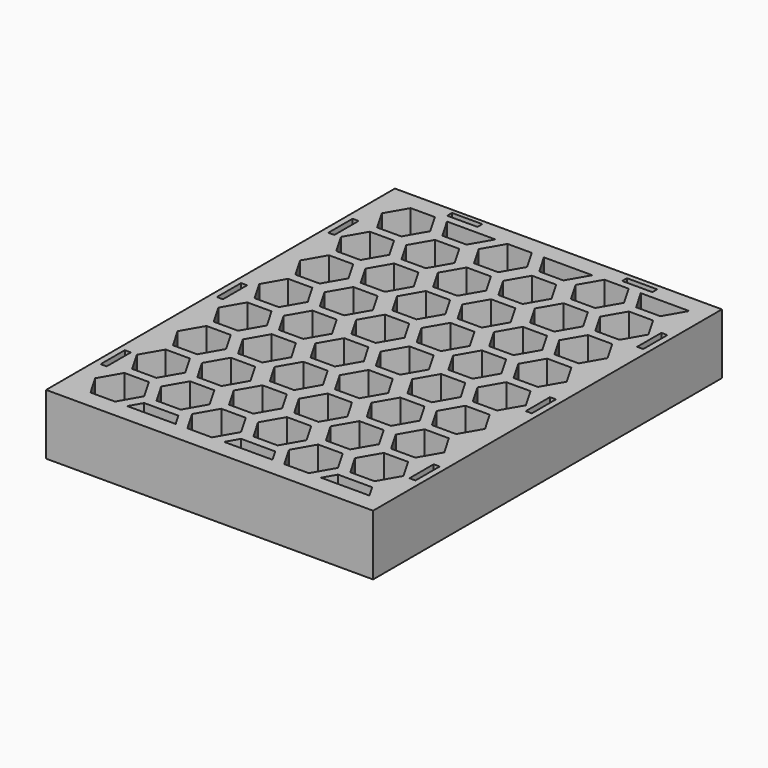
from build123d import *

# Parameters (mm, degrees)
F0_W     = 129.54
F0_H     = 179.07
F1_DEPTH = 25.4
F2_DEPTH = 25.4
F3_DEPTH = 25.4
F5_DEPTH = 25.4
F6_DEPTH = 25.4
F7_W     = 2.54
F7_H     = 12.7
F7_W_2   = 12.7
F7_H_2   = 2.54
F8_DEPTH = 7.62


# Not quite as in the source:
# - a feature names something its author has since deleted; it is built from what else it names


with BuildPart() as f1:
    # F0 (on Top) → F1 (new body)
    with BuildSketch(Plane.XY):
        with Locations((-1.3964310432, 21.6441547314)):
            Rectangle(F0_W, F0_H)
        Polygon((-62.5745659385, -51.3775706631), (-57.4400322633, -42.4842973522), (-47.1709648156, -42.484297296), (-42.0364310432, -51.3775705508), (-47.1709647184, -60.2708438618), (-57.440032166, -60.2708439179), align=None, mode=Mode.SUBTRACT)
        Polygon((-42.0364310432, -60.2708453796), (-39.0470681494, -55.0931169001), (-24.7057939935, -55.0931168217), (-21.7164310432, -60.2708452686), align=None, mode=Mode.SUBTRACT)
        Polygon((-21.9345659385, -51.3775720702), (-16.8000322633, -42.4842987593), (-6.5309648156, -42.4842987032), (-1.3964310432, -51.377571958), (-6.5309647184, -60.2708452689), (-16.800032166, -60.270845325), align=None, mode=Mode.SUBTRACT)
        Polygon((-42.0364310432, -42.4842988139), (-36.9564310912, -33.6854806837), (-26.7964310912, -33.6854806282), (-21.7164310432, -42.4842987029), (-26.7964309951, -51.2831168331), (-36.9564309951, -51.2831168886), align=None, mode=Mode.SUBTRACT)
        Polygon((-21.7164310432, -29.8754806837), (-16.6364310912, -21.0766625535), (-6.4764310912, -21.076662498), (-1.3964310432, -29.8754805727), (-6.4764309951, -38.6742987029), (-16.6364309951, -38.6742987584), align=None, mode=Mode.SUBTRACT)
        Polygon((-42.0364310432, -21.076662609), (-36.9564310912, -12.2778444788), (-26.7964310912, -12.2778444233), (-21.7164310432, -21.076662498), (-26.7964309951, -29.8754806282), (-36.9564309951, -29.8754806837), align=None, mode=Mode.SUBTRACT)
        Polygon((-42.0364310432, 0.3309735959), (-36.9564310912, 9.1297917261), (-26.7964310912, 9.1297917816), (-21.7164310432, 0.3309737069), (-26.7964309951, -8.4678444233), (-36.9564309951, -8.4678444788), align=None, mode=Mode.SUBTRACT)
        Polygon((-21.7164310432, -8.4678444788), (-16.6364310912, 0.3309736514), (-6.4764310912, 0.3309737069), (-1.3964310432, -8.4678443678), (-6.4764309951, -17.266662498), (-16.6364309951, -17.2666625535), align=None, mode=Mode.SUBTRACT)
        Polygon((-42.0364310432, 21.7386098008), (-36.9564310912, 30.537427931), (-26.7964310912, 30.5374279865), (-21.7164310432, 21.7386099118), (-26.7964309951, 12.9397917816), (-36.9564309951, 12.9397917261), align=None, mode=Mode.SUBTRACT)
        Polygon((-21.7164310432, 12.9397917261), (-16.6364310912, 21.7386098563), (-6.4764310912, 21.7386099118), (-1.3964310432, 12.9397918371), (-6.4764309951, 4.1409737069), (-16.6364309951, 4.1409736514), align=None, mode=Mode.SUBTRACT)
        Polygon((-1.3964310432, -60.2708452686), (1.5929318789, -55.0931168053), (15.9342060348, -55.0931168053), (18.9235689568, -60.2708452686), align=None, mode=Mode.SUBTRACT)
        Polygon((18.7054340615, -51.3775719857), (23.8399677854, -42.4842987029), (34.109035233, -42.4842987029), (39.2435689568, -51.3775719857), (34.109035233, -60.2708452686), (23.8399677854, -60.2708452686), align=None, mode=Mode.SUBTRACT)
        Polygon((-1.3964310432, -42.4842987029), (3.6835689568, -33.6854806004), (13.8435689568, -33.6854806004), (18.9235689568, -42.4842987029), (13.8435689568, -51.2831168053), (3.6835689568, -51.2831168053), align=None, mode=Mode.SUBTRACT)
        Polygon((18.9235689568, -29.8754806004), (24.0035689568, -21.076662498), (34.1635689568, -21.076662498), (39.2435689568, -29.8754806004), (34.1635689568, -38.6742987029), (24.0035689568, -38.6742987029), align=None, mode=Mode.SUBTRACT)
        Polygon((39.2435689568, -60.2708452686), (42.2329318789, -55.0931168053), (56.5742060348, -55.0931168053), (59.5635689568, -60.2708452686), align=None, mode=Mode.SUBTRACT)
        Polygon((-1.3964310432, -21.076662498), (3.6835689568, -12.2778443955), (13.8435689568, -12.2778443955), (18.9235689568, -21.076662498), (13.8435689568, -29.8754806004), (3.6835689568, -29.8754806004), align=None, mode=Mode.SUBTRACT)
        Polygon((-1.3964310432, 0.3309737069), (3.6835689568, 9.1297918094), (13.8435689568, 9.1297918094), (18.9235689568, 0.3309737069), (13.8435689568, -8.4678443955), (3.6835689568, -8.4678443955), align=None, mode=Mode.SUBTRACT)
        Polygon((18.9235689568, -8.4678443955), (24.0035689568, 0.3309737069), (34.1635689568, 0.3309737069), (39.2435689568, -8.4678443955), (34.1635689568, -17.266662498), (24.0035689568, -17.266662498), align=None, mode=Mode.SUBTRACT)
        Polygon((-1.3964310432, 21.7386099118), (3.6835689568, 30.5374280143), (13.8435689568, 30.5374280143), (18.9235689568, 21.7386099118), (13.8435689568, 12.9397918094), (3.6835689568, 12.9397918094), align=None, mode=Mode.SUBTRACT)
        Polygon((18.9235689568, 12.9397918094), (24.0035689568, 21.7386099118), (34.1635689568, 21.7386099118), (39.2435689568, 12.9397918094), (34.1635689568, 4.1409737069), (24.0035689568, 4.1409737069), align=None, mode=Mode.SUBTRACT)
        Polygon((-42.0364310432, 43.1462460057), (-36.9564310912, 51.9450641359), (-26.7964310912, 51.9450641914), (-21.7164310432, 43.1462461167), (-26.7964309951, 34.3474279865), (-36.9564309951, 34.347427931), align=None, mode=Mode.SUBTRACT)
        Polygon((-21.7164310432, 34.347427931), (-16.6364310912, 43.1462460612), (-6.4764310912, 43.1462461167), (-1.3964310432, 34.347428042), (-6.4764309951, 25.5486099118), (-16.6364309951, 25.5486098563), align=None, mode=Mode.SUBTRACT)
        Polygon((-42.0364310432, 64.5538822106), (-36.9564310912, 73.3527003408), (-26.7964310912, 73.3527003963), (-21.7164310432, 64.5538823216), (-26.7964309951, 55.7550641914), (-36.9564309951, 55.7550641359), align=None, mode=Mode.SUBTRACT)
        Polygon((-21.7164310432, 55.7550641359), (-16.6364310912, 64.5538822661), (-6.4764310912, 64.5538823216), (-1.3964310432, 55.7550642469), (-6.4764309951, 46.9562461167), (-16.6364309951, 46.9562460612), align=None, mode=Mode.SUBTRACT)
        Polygon((-62.3564310432, 98.5703361507), (-57.2764318716, 107.3691547314), (-47.1164318716, 107.369155688), (-42.0364310432, 98.5703380639), (-47.1164302147, 89.7715194831), (-57.2764302147, 89.7715185265), align=None, mode=Mode.SUBTRACT)
        Polygon((-42.0364310432, 85.9615184155), (-36.9564310912, 94.7603365457), (-26.7964310912, 94.7603366012), (-21.7164310432, 85.9615185265), (-26.7964309951, 77.1627003963), (-36.9564309951, 77.1627003408), align=None, mode=Mode.SUBTRACT)
        Polygon((-21.7164310432, 77.1627003408), (-16.6364310912, 85.961518471), (-6.4764310912, 85.9615185265), (-1.3964310432, 77.1627004518), (-6.4764309951, 68.3638823216), (-16.6364309951, 68.3638822661), align=None, mode=Mode.SUBTRACT)
        Polygon((-36.9564309951, 98.5703365457), (-42.0364310432, 107.3691546204), (-21.7164310432, 107.3691547314), (-26.7964309951, 98.5703366012), align=None, mode=Mode.SUBTRACT)
        Polygon((-21.7164310432, 98.5703365457), (-16.6364310912, 107.3691546759), (-6.4764310912, 107.3691547314), (-1.3964310432, 98.5703366567), (-6.4764309951, 89.7715185265), (-16.6364309951, 89.771518471), align=None, mode=Mode.SUBTRACT)
        Polygon((-1.3964310432, 43.1462461167), (3.6835689568, 51.9450642192), (13.8435689568, 51.9450642192), (18.9235689568, 43.1462461167), (13.8435689568, 34.3474280143), (3.6835689568, 34.3474280143), align=None, mode=Mode.SUBTRACT)
        Polygon((18.9235689568, 34.3474280143), (24.0035689568, 43.1462461167), (34.1635689568, 43.1462461167), (39.2435689568, 34.3474280143), (34.1635689568, 25.5486099118), (24.0035689568, 25.5486099118), align=None, mode=Mode.SUBTRACT)
        Polygon((-1.3964310432, 64.5538823216), (3.6835689568, 73.3527004241), (13.8435689568, 73.3527004241), (18.9235689568, 64.5538823216), (13.8435689568, 55.7550642192), (3.6835689568, 55.7550642192), align=None, mode=Mode.SUBTRACT)
        Polygon((18.9235689568, 55.7550642192), (24.0035689568, 64.5538823216), (34.1635689568, 64.5538823216), (39.2435689568, 55.7550642192), (34.1635689568, 46.9562461167), (24.0035689568, 46.9562461167), align=None, mode=Mode.SUBTRACT)
        Polygon((-1.3964310432, 85.9615185265), (3.6835689568, 94.760336629), (13.8435689568, 94.760336629), (18.9235689568, 85.9615185265), (13.8435689568, 77.1627004241), (3.6835689568, 77.1627004241), align=None, mode=Mode.SUBTRACT)
        Polygon((18.9235689568, 77.1627004241), (24.0035689568, 85.9615185265), (34.1635689568, 85.9615185265), (39.2435689568, 77.1627004241), (34.1635689568, 68.3638823216), (24.0035689568, 68.3638823216), align=None, mode=Mode.SUBTRACT)
        Polygon((3.6835689568, 98.570336629), (-1.3964310432, 107.3691547314), (18.9235689568, 107.3691547314), (13.8435689568, 98.570336629), align=None, mode=Mode.SUBTRACT)
        Polygon((18.9235689568, 98.570336629), (24.0035689568, 107.3691547314), (34.1635689568, 107.3691547314), (39.2435689568, 98.570336629), (34.1635689568, 89.7715185265), (24.0035689568, 89.7715185265), align=None, mode=Mode.SUBTRACT)
        Polygon((44.3235689568, 98.570336629), (39.2435689568, 107.3691547314), (59.5635689568, 107.3691547314), (54.4835689568, 98.570336629), align=None, mode=Mode.SUBTRACT)
        Polygon((34.109035233, -42.4842987029), (23.8399677854, -42.4842987029), (18.7054340615, -51.3775719857), (23.8399677854, -60.2708452686), (34.109035233, -60.2708452686), (39.2435689568, -51.3775719857), align=None)
        Polygon((-6.5309648156, -42.4842987032), (-16.8000322633, -42.4842987593), (-21.9345659385, -51.3775720702), (-16.800032166, -60.270845325), (-6.5309647184, -60.2708452689), (-1.3964310432, -51.377571958), align=None)
        Polygon((-47.1709648156, -42.484297296), (-57.4400322633, -42.4842973522), (-62.5745659385, -51.3775706631), (-57.440032166, -60.2708439179), (-47.1709647184, -60.2708438618), (-42.0364310432, -51.3775705508), align=None)
        Polygon((-26.7964310912, 51.9450641914), (-36.9564310912, 51.9450641359), (-42.0364310432, 43.1462460057), (-36.9564309951, 34.347427931), (-26.7964309951, 34.3474279865), (-21.7164310432, 43.1462461167), align=None)
        Polygon((-6.4764310912, 43.1462461167), (-16.6364310912, 43.1462460612), (-21.7164310432, 34.347427931), (-16.6364309951, 25.5486098563), (-6.4764309951, 25.5486099118), (-1.3964310432, 34.347428042), align=None)
        Polygon((-6.4764310912, 21.7386099118), (-16.6364310912, 21.7386098563), (-21.7164310432, 12.9397917261), (-16.6364309951, 4.1409736514), (-6.4764309951, 4.1409737069), (-1.3964310432, 12.9397918371), align=None)
        Polygon((-6.4764310912, 0.3309737069), (-16.6364310912, 0.3309736514), (-21.7164310432, -8.4678444788), (-16.6364309951, -17.2666625535), (-6.4764309951, -17.266662498), (-1.3964310432, -8.4678443678), align=None)
        Polygon((-26.7964310912, -12.2778444233), (-36.9564310912, -12.2778444788), (-42.0364310432, -21.076662609), (-36.9564309951, -29.8754806837), (-26.7964309951, -29.8754806282), (-21.7164310432, -21.076662498), align=None)
        Polygon((-6.4764310912, -21.076662498), (-16.6364310912, -21.0766625535), (-21.7164310432, -29.8754806837), (-16.6364309951, -38.6742987584), (-6.4764309951, -38.6742987029), (-1.3964310432, -29.8754805727), align=None)
        Polygon((-26.7964310912, -33.6854806282), (-36.9564310912, -33.6854806837), (-42.0364310432, -42.4842988139), (-36.9564309951, -51.2831168886), (-26.7964309951, -51.2831168331), (-21.7164310432, -42.4842987029), align=None)
        Polygon((13.8435689568, -12.2778443955), (3.6835689568, -12.2778443955), (-1.3964310432, -21.076662498), (3.6835689568, -29.8754806004), (13.8435689568, -29.8754806004), (18.9235689568, -21.076662498), align=None)
        Polygon((13.8435689568, 9.1297918094), (3.6835689568, 9.1297918094), (-1.3964310432, 0.3309737069), (3.6835689568, -8.4678443955), (13.8435689568, -8.4678443955), (18.9235689568, 0.3309737069), align=None)
        Polygon((34.1635689568, 0.3309737069), (24.0035689568, 0.3309737069), (18.9235689568, -8.4678443955), (24.0035689568, -17.266662498), (34.1635689568, -17.266662498), (39.2435689568, -8.4678443955), align=None)
        Polygon((34.1635689568, -21.076662498), (24.0035689568, -21.076662498), (18.9235689568, -29.8754806004), (24.0035689568, -38.6742987029), (34.1635689568, -38.6742987029), (39.2435689568, -29.8754806004), align=None)
        Polygon((34.1635689568, 21.7386099118), (24.0035689568, 21.7386099118), (18.9235689568, 12.9397918094), (24.0035689568, 4.1409737069), (34.1635689568, 4.1409737069), (39.2435689568, 12.9397918094), align=None)
        Polygon((13.8435689568, 30.5374280143), (3.6835689568, 30.5374280143), (-1.3964310432, 21.7386099118), (3.6835689568, 12.9397918094), (13.8435689568, 12.9397918094), (18.9235689568, 21.7386099118), align=None)
        Polygon((34.1635689568, 43.1462461167), (24.0035689568, 43.1462461167), (18.9235689568, 34.3474280143), (24.0035689568, 25.5486099118), (34.1635689568, 25.5486099118), (39.2435689568, 34.3474280143), align=None)
        Polygon((13.8435689568, 51.9450642192), (3.6835689568, 51.9450642192), (-1.3964310432, 43.1462461167), (3.6835689568, 34.3474280143), (13.8435689568, 34.3474280143), (18.9235689568, 43.1462461167), align=None)
        Polygon((34.1635689568, 64.5538823216), (24.0035689568, 64.5538823216), (18.9235689568, 55.7550642192), (24.0035689568, 46.9562461167), (34.1635689568, 46.9562461167), (39.2435689568, 55.7550642192), align=None)
        Polygon((13.8435689568, 73.3527004241), (3.6835689568, 73.3527004241), (-1.3964310432, 64.5538823216), (3.6835689568, 55.7550642192), (13.8435689568, 55.7550642192), (18.9235689568, 64.5538823216), align=None)
        Polygon((-6.4764310912, 64.5538823216), (-16.6364310912, 64.5538822661), (-21.7164310432, 55.7550641359), (-16.6364309951, 46.9562460612), (-6.4764309951, 46.9562461167), (-1.3964310432, 55.7550642469), align=None)
        Polygon((-26.7964310912, 73.3527003963), (-36.9564310912, 73.3527003408), (-42.0364310432, 64.5538822106), (-36.9564309951, 55.7550641359), (-26.7964309951, 55.7550641914), (-21.7164310432, 64.5538823216), align=None)
        Polygon((-26.7964310912, 94.7603366012), (-36.9564310912, 94.7603365457), (-42.0364310432, 85.9615184155), (-36.9564309951, 77.1627003408), (-26.7964309951, 77.1627003963), (-21.7164310432, 85.9615185265), align=None)
        Polygon((-6.4764310912, 85.9615185265), (-16.6364310912, 85.961518471), (-21.7164310432, 77.1627003408), (-16.6364309951, 68.3638822661), (-6.4764309951, 68.3638823216), (-1.3964310432, 77.1627004518), align=None)
        Polygon((13.8435689568, 94.760336629), (3.6835689568, 94.760336629), (-1.3964310432, 85.9615185265), (3.6835689568, 77.1627004241), (13.8435689568, 77.1627004241), (18.9235689568, 85.9615185265), align=None)
        Polygon((34.1635689568, 85.9615185265), (24.0035689568, 85.9615185265), (18.9235689568, 77.1627004241), (24.0035689568, 68.3638823216), (34.1635689568, 68.3638823216), (39.2435689568, 77.1627004241), align=None)
        Polygon((13.8435689568, -33.6854806004), (3.6835689568, -33.6854806004), (-1.3964310432, -42.4842987029), (3.6835689568, -51.2831168053), (13.8435689568, -51.2831168053), (18.9235689568, -42.4842987029), align=None)
        Polygon((-47.1164318716, 107.369155688), (-57.2764318716, 107.3691547314), (-62.3564310432, 98.5703361507), (-57.2764302147, 89.7715185265), (-47.1164302147, 89.7715194831), (-42.0364310432, 98.5703380639), align=None)
        Polygon((34.1635689568, 107.3691547314), (24.0035689568, 107.3691547314), (18.9235689568, 98.570336629), (24.0035689568, 89.7715185265), (34.1635689568, 89.7715185265), (39.2435689568, 98.570336629), align=None)
        Polygon((-21.7164310432, 107.3691547314), (-42.0364310432, 107.3691546204), (-36.9564309951, 98.5703365457), (-26.7964309951, 98.5703366012), align=None)
        Polygon((59.5635689568, 107.3691547314), (39.2435689568, 107.3691547314), (44.3235689568, 98.570336629), (54.4835689568, 98.570336629), align=None)
        Polygon((56.5742060348, -55.0931168053), (42.2329318789, -55.0931168053), (39.2435689568, -60.2708452686), (59.5635689568, -60.2708452686), align=None)
        Polygon((15.9342060348, -55.0931168053), (1.5929318789, -55.0931168053), (-1.3964310432, -60.2708452686), (18.9235689568, -60.2708452686), align=None)
        Polygon((-24.7057939935, -55.0931168217), (-39.0470681494, -55.0931169001), (-42.0364310432, -60.2708453796), (-21.7164310432, -60.2708452686), align=None)
    extrude(amount=F1_DEPTH)

    # F0 (on Top) → F2 (cut)
    with BuildSketch(Plane.XY):
        Polygon((-6.4764310912, -21.076662498), (-16.6364310912, -21.0766625535), (-21.7164310432, -29.8754806837), (-16.6364309951, -38.6742987584), (-6.4764309951, -38.6742987029), (-1.3964310432, -29.8754805727), align=None)
        Polygon((-26.7964310912, -12.2778444233), (-36.9564310912, -12.2778444788), (-42.0364310432, -21.076662609), (-36.9564309951, -29.8754806837), (-26.7964309951, -29.8754806282), (-21.7164310432, -21.076662498), align=None)
        Polygon((-26.7964310912, -33.6854806282), (-36.9564310912, -33.6854806837), (-42.0364310432, -42.4842988139), (-36.9564309951, -51.2831168886), (-26.7964309951, -51.2831168331), (-21.7164310432, -42.4842987029), align=None)
        Polygon((-6.4764310912, 0.3309737069), (-16.6364310912, 0.3309736514), (-21.7164310432, -8.4678444788), (-16.6364309951, -17.2666625535), (-6.4764309951, -17.266662498), (-1.3964310432, -8.4678443678), align=None)
        Polygon((-6.4764310912, 21.7386099118), (-16.6364310912, 21.7386098563), (-21.7164310432, 12.9397917261), (-16.6364309951, 4.1409736514), (-6.4764309951, 4.1409737069), (-1.3964310432, 12.9397918371), align=None)
        Polygon((-6.4764310912, 43.1462461167), (-16.6364310912, 43.1462460612), (-21.7164310432, 34.347427931), (-16.6364309951, 25.5486098563), (-6.4764309951, 25.5486099118), (-1.3964310432, 34.347428042), align=None)
        Polygon((-6.4764310912, 64.5538823216), (-16.6364310912, 64.5538822661), (-21.7164310432, 55.7550641359), (-16.6364309951, 46.9562460612), (-6.4764309951, 46.9562461167), (-1.3964310432, 55.7550642469), align=None)
        Polygon((-6.4764310912, 85.9615185265), (-16.6364310912, 85.961518471), (-21.7164310432, 77.1627003408), (-16.6364309951, 68.3638822661), (-6.4764309951, 68.3638823216), (-1.3964310432, 77.1627004518), align=None)
        Polygon((13.8435689568, 94.760336629), (3.6835689568, 94.760336629), (-1.3964310432, 85.9615185265), (3.6835689568, 77.1627004241), (13.8435689568, 77.1627004241), (18.9235689568, 85.9615185265), align=None)
        Polygon((13.8435689568, 73.3527004241), (3.6835689568, 73.3527004241), (-1.3964310432, 64.5538823216), (3.6835689568, 55.7550642192), (13.8435689568, 55.7550642192), (18.9235689568, 64.5538823216), align=None)
        Polygon((13.8435689568, 51.9450642192), (3.6835689568, 51.9450642192), (-1.3964310432, 43.1462461167), (3.6835689568, 34.3474280143), (13.8435689568, 34.3474280143), (18.9235689568, 43.1462461167), align=None)
        Polygon((13.8435689568, 30.5374280143), (3.6835689568, 30.5374280143), (-1.3964310432, 21.7386099118), (3.6835689568, 12.9397918094), (13.8435689568, 12.9397918094), (18.9235689568, 21.7386099118), align=None)
        Polygon((13.8435689568, 9.1297918094), (3.6835689568, 9.1297918094), (-1.3964310432, 0.3309737069), (3.6835689568, -8.4678443955), (13.8435689568, -8.4678443955), (18.9235689568, 0.3309737069), align=None)
        Polygon((13.8435689568, -12.2778443955), (3.6835689568, -12.2778443955), (-1.3964310432, -21.076662498), (3.6835689568, -29.8754806004), (13.8435689568, -29.8754806004), (18.9235689568, -21.076662498), align=None)
        Polygon((13.8435689568, -33.6854806004), (3.6835689568, -33.6854806004), (-1.3964310432, -42.4842987029), (3.6835689568, -51.2831168053), (13.8435689568, -51.2831168053), (18.9235689568, -42.4842987029), align=None)
        Polygon((34.1635689568, -21.076662498), (24.0035689568, -21.076662498), (18.9235689568, -29.8754806004), (24.0035689568, -38.6742987029), (34.1635689568, -38.6742987029), (39.2435689568, -29.8754806004), align=None)
        Polygon((34.1635689568, 0.3309737069), (24.0035689568, 0.3309737069), (18.9235689568, -8.4678443955), (24.0035689568, -17.266662498), (34.1635689568, -17.266662498), (39.2435689568, -8.4678443955), align=None)
        Polygon((34.1635689568, 21.7386099118), (24.0035689568, 21.7386099118), (18.9235689568, 12.9397918094), (24.0035689568, 4.1409737069), (34.1635689568, 4.1409737069), (39.2435689568, 12.9397918094), align=None)
        Polygon((34.1635689568, 43.1462461167), (24.0035689568, 43.1462461167), (18.9235689568, 34.3474280143), (24.0035689568, 25.5486099118), (34.1635689568, 25.5486099118), (39.2435689568, 34.3474280143), align=None)
        Polygon((34.1635689568, 64.5538823216), (24.0035689568, 64.5538823216), (18.9235689568, 55.7550642192), (24.0035689568, 46.9562461167), (34.1635689568, 46.9562461167), (39.2435689568, 55.7550642192), align=None)
        Polygon((34.1635689568, 85.9615185265), (24.0035689568, 85.9615185265), (18.9235689568, 77.1627004241), (24.0035689568, 68.3638823216), (34.1635689568, 68.3638823216), (39.2435689568, 77.1627004241), align=None)
        Polygon((-26.7964310912, 51.9450641914), (-36.9564310912, 51.9450641359), (-42.0364310432, 43.1462460057), (-36.9564309951, 34.347427931), (-26.7964309951, 34.3474279865), (-21.7164310432, 43.1462461167), align=None)
        Polygon((-26.7964310912, 73.3527003963), (-36.9564310912, 73.3527003408), (-42.0364310432, 64.5538822106), (-36.9564309951, 55.7550641359), (-26.7964309951, 55.7550641914), (-21.7164310432, 64.5538823216), align=None)
        Polygon((-26.7964310912, 94.7603366012), (-36.9564310912, 94.7603365457), (-42.0364310432, 85.9615184155), (-36.9564309951, 77.1627003408), (-26.7964309951, 77.1627003963), (-21.7164310432, 85.9615185265), align=None)
    extrude(amount=F2_DEPTH, mode=Mode.SUBTRACT)

    # F0 (on Top) → F3 (cut)
    with BuildSketch(Plane.XY):
        Polygon((-24.7057939935, -55.0931168217), (-39.0470681494, -55.0931169001), (-42.0364310432, -60.2708453796), (-21.7164310432, -60.2708452686), align=None)
        Polygon((15.9342060348, -55.0931168053), (1.5929318789, -55.0931168053), (-1.3964310432, -60.2708452686), (18.9235689568, -60.2708452686), align=None)
        Polygon((56.5742060348, -55.0931168053), (42.2329318789, -55.0931168053), (39.2435689568, -60.2708452686), (59.5635689568, -60.2708452686), align=None)
        Polygon((59.5635689568, 107.3691547314), (39.2435689568, 107.3691547314), (44.3235689568, 98.570336629), (54.4835689568, 98.570336629), align=None)
        Polygon((-21.7164310432, 107.3691547314), (-42.0364310432, 107.3691546204), (-36.9564309951, 98.5703365457), (-26.7964309951, 98.5703366012), align=None)
        Polygon((-6.5309648156, -42.4842987032), (-16.8000322633, -42.4842987593), (-21.9345659385, -51.3775720702), (-16.800032166, -60.270845325), (-6.5309647184, -60.2708452689), (-1.3964310432, -51.377571958), align=None)
        Polygon((34.109035233, -42.4842987029), (23.8399677854, -42.4842987029), (18.7054340615, -51.3775719857), (23.8399677854, -60.2708452686), (34.109035233, -60.2708452686), (39.2435689568, -51.3775719857), align=None)
        Polygon((34.1635689568, 107.3691547314), (24.0035689568, 107.3691547314), (18.9235689568, 98.570336629), (24.0035689568, 89.7715185265), (34.1635689568, 89.7715185265), (39.2435689568, 98.570336629), align=None)
        Polygon((-47.1164318716, 107.369155688), (-57.2764318716, 107.3691547314), (-62.3564310432, 98.5703361507), (-57.2764302147, 89.7715185265), (-47.1164302147, 89.7715194831), (-42.0364310432, 98.5703380639), align=None)
        Polygon((-47.1709648156, -42.484297296), (-57.4400322633, -42.4842973522), (-62.5745659385, -51.3775706631), (-57.440032166, -60.2708439179), (-47.1709647184, -60.2708438618), (-42.0364310432, -51.3775705508), align=None)
    extrude(amount=F3_DEPTH, mode=Mode.SUBTRACT)

    # F4 (on face) → F5 (cut)
    with BuildSketch(Plane.XY):
        Polygon((39.2435689568, -42.4842987029), (44.3235689568, -51.2831168053), (54.4835689568, -51.2831168053), (59.5635689568, -42.4842987029), (54.4835689568, -33.6854806004), (44.3235689568, -33.6854806004), align=None)
        Polygon((39.2435689568, -21.076662498), (44.3235689568, -29.8754806004), (54.4835689568, -29.8754806004), (59.5635689568, -21.076662498), (54.4835689568, -12.2778443955), (44.3235689568, -12.2778443955), align=None)
        Polygon((39.2435689568, 0.3309737069), (44.3235689568, -8.4678443955), (54.4835689568, -8.4678443955), (59.5635689568, 0.3309737069), (54.4835689568, 9.1297918094), (44.3235689568, 9.1297918094), align=None)
        Polygon((39.2435689568, 21.7386099118), (44.3235689568, 12.9397918094), (54.4835689568, 12.9397918094), (59.5635689568, 21.7386099118), (54.4835689568, 30.5374280143), (44.3235689568, 30.5374280143), align=None)
        Polygon((39.2435689568, 43.1462461167), (44.3235689568, 34.3474280143), (54.4835689568, 34.3474280143), (59.5635689568, 43.1462461167), (54.4835689568, 51.9450642192), (44.3235689568, 51.9450642192), align=None)
        Polygon((39.2435689568, 64.5538823216), (44.3235689568, 55.7550642192), (54.4835689568, 55.7550642192), (59.5635689568, 64.5538823216), (54.4835689568, 73.3527004241), (44.3235689568, 73.3527004241), align=None)
        Polygon((39.2435689568, 85.9615185265), (44.3235689568, 77.1627004241), (54.4835689568, 77.1627004241), (59.5635689568, 85.9615185265), (54.4835689568, 94.760336629), (44.3235689568, 94.760336629), align=None)
        Polygon((-62.3564310432, 77.1627017479), (-57.2764309951, 68.3638836732), (-47.1164309951, 68.3638837287), (-42.0364310432, 77.162701859), (-47.1164310912, 85.9615199336), (-57.2764310912, 85.9615198781), align=None)
        Polygon((-62.3564310432, 55.755065543), (-57.2764309951, 46.9562474683), (-47.1164309951, 46.9562475238), (-42.0364310432, 55.7550656541), (-47.1164310912, 64.5538837287), (-57.2764310912, 64.5538836732), align=None)
        Polygon((-62.3564310432, 34.3474293381), (-57.2764309951, 25.5486112634), (-47.1164309951, 25.5486113189), (-42.0364310432, 34.3474294492), (-47.1164310912, 43.1462475238), (-57.2764310912, 43.1462474683), align=None)
        Polygon((-62.3564310432, 12.9397931332), (-57.2764309951, 4.1409750585), (-47.1164309951, 4.140975114), (-42.0364310432, 12.9397932443), (-47.1164310912, 21.7386113189), (-57.2764310912, 21.7386112634), align=None)
        Polygon((-62.3564310432, -8.4678430717), (-57.2764309951, -17.2666611464), (-47.1164309951, -17.2666610909), (-42.0364310432, -8.4678429606), (-47.1164310912, 0.330975114), (-57.2764310912, 0.3309750585), align=None)
        Polygon((-62.3564310432, -29.8754792766), (-57.2764309951, -38.6742973513), (-47.1164309951, -38.6742972958), (-42.0364310432, -29.8754791655), (-47.1164310912, -21.0766610909), (-57.2764310912, -21.0766611464), align=None)
    extrude(amount=F5_DEPTH, mode=Mode.SUBTRACT)

    # F0 (on Top) → F6 (join)
    with BuildSketch(Plane.XY):
        Polygon((67.1835689568, 114.9891547314), (-69.9764310432, 114.9891547314), (-69.9764310432, -67.8908452686), (-66.1664310432, -67.8908452686), (-66.1664310432, 111.1791547314), (63.3735689568, 111.1791547314), (63.3735689568, -67.8908452686), (67.1835689568, -67.8908452686), align=None)
    extrude(amount=F6_DEPTH)

    # F7 (on face) → F8 (cut)
    with BuildSketch(Plane.XY.offset(25.4)):
        with Locations((-66.1664310432, -36.1408452686)):
            Rectangle(F7_W, F7_H)
        with Locations((-66.1664310432, 24.8191547314)):
            Rectangle(F7_W, F7_H)
        with Locations((63.3735689568, -36.1408452686)):
            Rectangle(F7_W, F7_H)
        with Locations((63.3735689568, 24.8191547314)):
            Rectangle(F7_W, F7_H)
        with Locations((63.3735689568, 83.2391547314)):
            Rectangle(F7_W, F7_H)
        with Locations((-66.1664310432, 83.2391547314)):
            Rectangle(F7_W, F7_H)
        with Locations((-38.2264310432, 111.8977257204)):
            Rectangle(F7_W_2, F7_H_2)
        with Locations((35.4335689568, 111.5483605456)):
            Rectangle(F7_W_2, F7_H_2)
    extrude(amount=-F8_DEPTH, mode=Mode.SUBTRACT)


solid = f1.part
